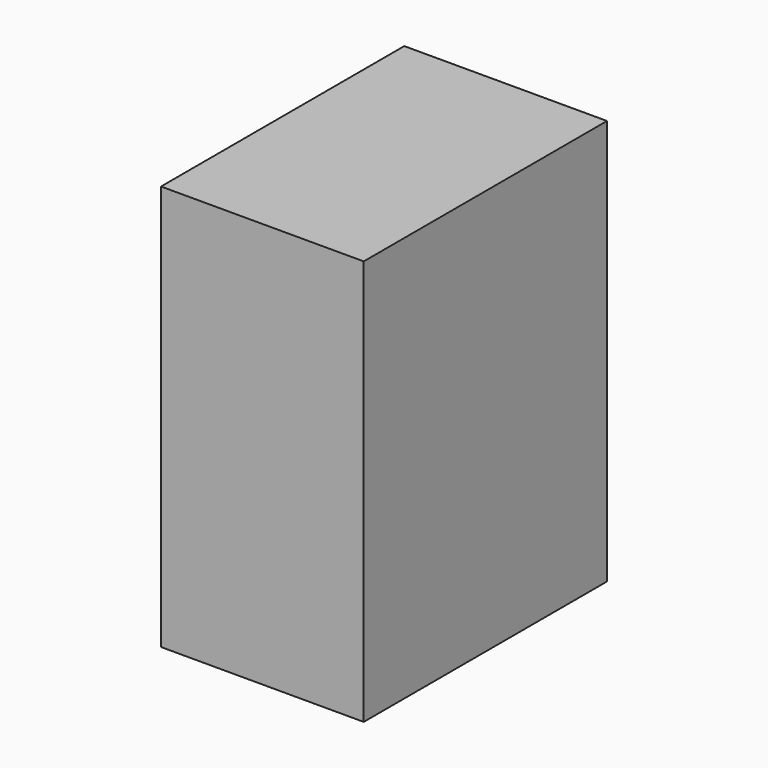
from build123d import *

# Parameters (mm, degrees)
F2_W     = 20
F2_H     = 30
F3_DEPTH = 40


# Not quite as in the source:
# - the program builds the solid bodies; features that only make, move or delete a surface that nothing else refers to are left out


with BuildPart() as f3:
    # F2 (on Top) → F3 (new body)
    with BuildSketch(Plane.XY):
        with Locations((10, 15)):
            Rectangle(F2_W, F2_H)
    extrude(amount=F3_DEPTH)


solid = f3.part
